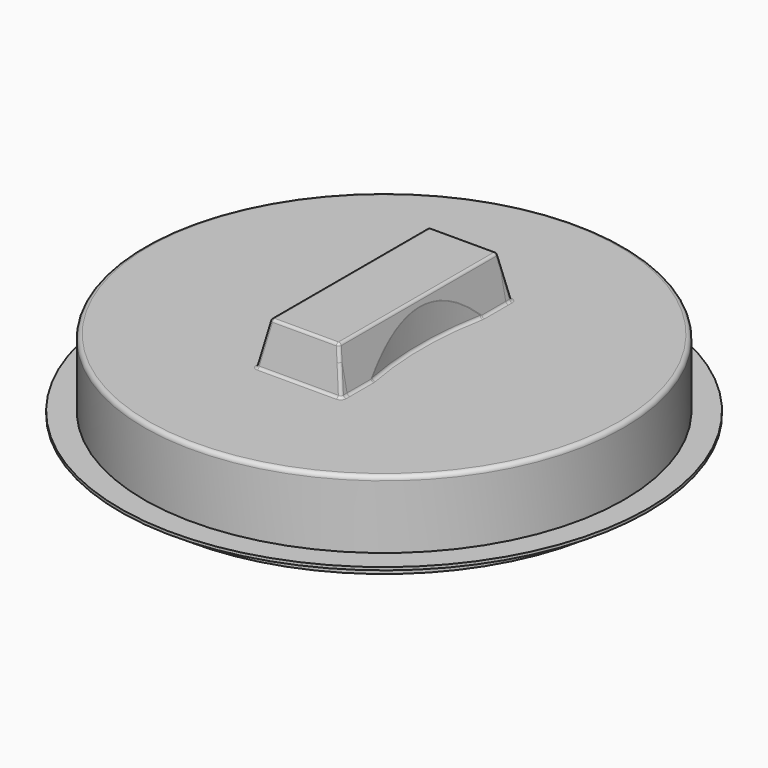
from build123d import *

# Parameters (mm, degrees)
F0_R      = 168.25
F0_R_2    = 167.5
F1_DEPTH  = 11
F0_R_3    = 185
F2_DEPTH  = 2
F3_DEPTH  = 47.5
F4_R      = 168.25
F4_R_2    = 167.5
F5_DEPTH  = 2
F6_R      = 3
F7_W      = 48
F7_H      = 139
F8_DEPTH  = 30
F10_DEPTH = 139
F15_R     = 250
F16_DEPTH = 30
F17_R     = 2


with BuildPart() as f1:
    # F0 (on Top) → F1 (new body)
    with BuildSketch(Plane.XY):
        Circle(F0_R)
        Circle(F0_R_2, mode=Mode.SUBTRACT)
    extrude(amount=-F1_DEPTH)

    # F0 (on Top) → F2 (join)
    with BuildSketch(Plane.XY):
        Circle(F0_R_3)
        Circle(F0_R, mode=Mode.SUBTRACT)
        Circle(F0_R)
        Circle(F0_R_2, mode=Mode.SUBTRACT)
    extrude(amount=F2_DEPTH)

    # F0 (on Top) → F3 (join)
    with BuildSketch(Plane.XY):
        Circle(F0_R)
        Circle(F0_R_2, mode=Mode.SUBTRACT)
    extrude(amount=F3_DEPTH)

    # F4 (on face) → F5 (join)
    with BuildSketch(Plane.XY.offset(47.5)):
        Circle(F4_R)
        Circle(F4_R_2, mode=Mode.SUBTRACT)
        Circle(F4_R_2)
    extrude(amount=F5_DEPTH)

    # F6
    f6_edges = [f1.edges().sort_by_distance(p)[0] for p in [
        (-168.25, 0, 49.5),
    ]]
    fillet(f6_edges, radius=F6_R)

    # F7 (on face) → F8 (join)
    with BuildSketch(Plane.XY.offset(49.5)):
        Rectangle(F7_W, F7_H)
    extrude(amount=F8_DEPTH)

    # F9 (on face) → F10 (join, through all)
    with BuildSketch(Plane.XZ.offset(69.5)):
        Polygon((-24, 49.5), (-24, 79.5), (-30, 49.5), align=None)
        Polygon((30, 49.5), (24, 79.5), (24, 49.5), align=None)
    extrude(amount=-F10_DEPTH)

    # F12: sweep along a path in F12_path
    with BuildLine(Plane(origin=(-24, 69.5, 79.5), x_dir=(0, 1, 0), z_dir=(0, 0, 1))) as f12_path:
        Line((0, 0), (0, -48))
    # F11 (on face) → F12 (sweep)
    with BuildSketch(Plane(origin=(-38.3653846154, 0, 7.6730769231), x_dir=(0, -1, 0), z_dir=(-0.9805806757, 0, 0.1961161351))):
        Polygon((-69.5, 42.6552593926), (-69.5, 73.2493764741), (-75, 42.6552593926), align=None)
        Polygon((75, 42.6552593926), (69.5, 73.2493764741), (69.5, 42.6552593926), align=None)
    sweep(path=f12_path.line)

    # F14: sweep along a path in F14_path
    with BuildLine(Plane(origin=(-24, 69.5, 79.5), x_dir=(0, 1, 0), z_dir=(0, 0, 1))) as f14_path:
        Line((0, 0), (0, -48))
    # F13 (on face) → F14 (sweep)
    with BuildSketch(Plane(origin=(38.3653846154, 0, 7.6730769231), x_dir=(0, 1, 0), z_dir=(0.9805806757, 0, 0.1961161351))):
        Polygon((75, 42.6552593926), (69.5, 73.2493764741), (69.5, 42.6552593926), align=None)
        Polygon((-69.5, 42.6552593926), (-69.5, 73.2493764741), (-75, 42.6552593926), align=None)
    sweep(path=f14_path.line)

    # F15 (on face) → F16 (cut, through all)
    with BuildSketch(Plane.XY.offset(79.5)):
        with Locations((-275, 0)):
            Circle(F15_R)
        with Locations((275, 0)):
            Circle(F15_R)
    extrude(amount=-F16_DEPTH, mode=Mode.SUBTRACT)

    # F17
    f17_edges = [f1.edges().sort_by_distance(p)[0] for p in [
        (0, -69.5, 79.5),
        (-24, 0, 79.5),
        (-26.501542, -27.359029, 66.992289),
        (-26.501542, 27.359029, 66.992289),
        (24, 0, 79.5),
        (0, 69.5, 79.5),
        (25, 0, 74.5),
        (25, 0, 49.5),
        (-25, 0, 49.5),
        (-30, -62.374686, 49.5),
        (-30, 62.374686, 49.5),
        (0, 75, 49.5),
        (30, 62.374686, 49.5),
        (30, -62.374686, 49.5),
        (0, -75, 49.5),
        (-27, -72.25, 64.5),
        (27, -72.25, 64.5),
        (27, 72.25, 64.5),
        (-27, 72.25, 64.5),
    ]]
    fillet(f17_edges, radius=F17_R)


solid = f1.part
